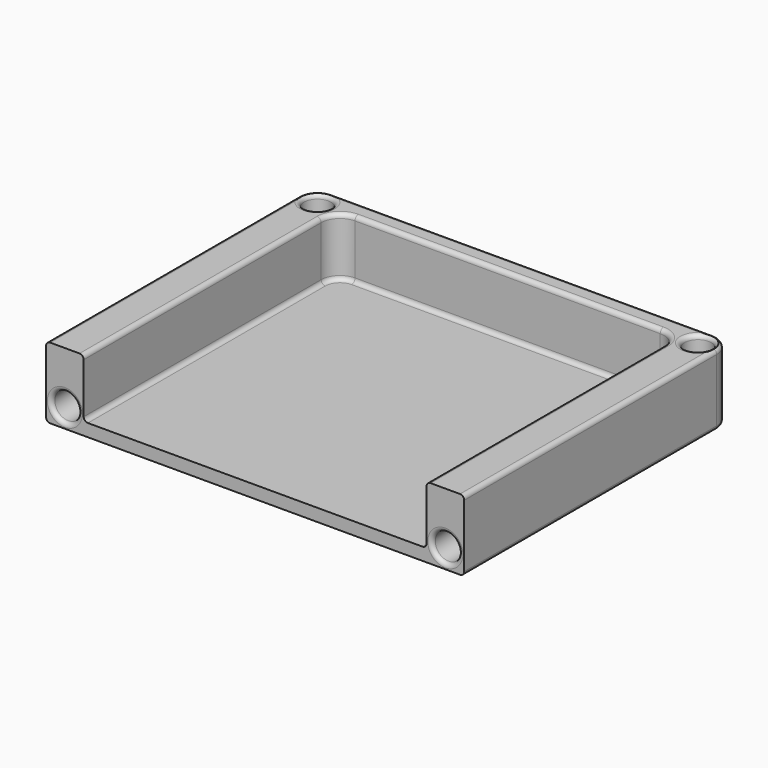
from build123d import *

# Parameters (mm, degrees)
F1_DEPTH     = 17
F5_DEPTH     = 14
F3_R         = 3.2
F6_DEPTH     = 10
F4_R         = 3.2
F7_DEPTH     = 10
F8_T1_DEPTH  = 73
F8_T3_DEPTH  = 71
F8_T6_ANGLE  = 90
F8_T8_ANGLE  = 90
F8_T9_DEPTH  = 78
F8_T11_DEPTH = 73.5
F8_T13_DEPTH = 73
F8_T15_DEPTH = 91
F8_T26_ANGLE = 90
F8_T28_ANGLE = 90
F8_T30_ANGLE = 90
F8_T32_ANGLE = 90
F8_T34_ANGLE = 90
F8_T36_ANGLE = 90


# Not quite as in the source:
# - a fillet or chamfer that OpenCascade refuses, or shapes differently, is made with other operations: its cross-section is extruded or revolved along the edge and cut away or added


with BuildPart() as f1:
    # F0 (on Top) → F1 (new body)
    with BuildSketch(Plane.XY):
        with BuildLine():
            Line((0, 75.5), (0, 0))
            Line((0, 0), (50, 0))
            Line((50, 0), (100, 0))
            Line((100, 0), (100, 75.5))
            ThreePointArc((100, 75.5), (98.6819805153, 78.6819805153), (95.5, 80))
            Line((95.5, 80), (50, 80))
            Line((50, 80), (4.5, 80))
            ThreePointArc((4.5, 80), (1.3180194847, 78.6819805153), (0, 75.5))
        make_face()
    extrude(amount=F1_DEPTH)

    # F3 (on offset) → F5 (cut)
    with BuildSketch(Plane.XY.offset(17)):
        with BuildLine():
            Line((9, 71), (9, 0))
            Line((9, 0), (50, 0))
            Line((50, 0), (91, 0))
            Line((91, 0), (91, 71))
            ThreePointArc((91, 71), (89.6819805153, 74.1819805153), (86.5, 75.5))
            Line((86.5, 75.5), (50, 75.5))
            Line((50, 75.5), (13.5, 75.5))
            ThreePointArc((13.5, 75.5), (10.3180194847, 74.1819805153), (9, 71))
        make_face()
    extrude(amount=-F5_DEPTH, mode=Mode.SUBTRACT)

    # F3 (on offset) → F6 (cut)
    with BuildSketch(Plane.XY.offset(17)):
        with Locations((4.5, 75.5)):
            Circle(F3_R)
        with Locations((95.5, 75.5)):
            Circle(F3_R)
    extrude(amount=-F6_DEPTH, mode=Mode.SUBTRACT)

    # F4 (on Front) → F7 (cut)
    with BuildSketch(Plane.XZ):
        with Locations((4.5, 4.5)):
            Circle(F4_R)
        with Locations((95.5, 4.5)):
            Circle(F4_R)
    extrude(amount=-F7_DEPTH, mode=Mode.SUBTRACT)

    # F8: fillet of radius 1 on 8 edges, made by hand

    # F8_s2 → F8_t1 (join)
    with BuildSketch(Plane.YZ.offset(13.5)):
        with BuildLine():
            ThreePointArc((74.5, 3), (75.2071067812, 3.2928932188), (75.5, 4))
            Line((75.5, 4), (75.5, 3))
            Line((75.5, 3), (74.5, 3))
        make_face()
    extrude(amount=F8_T1_DEPTH)

    # F8_s4 → F8_t3 (join)
    with BuildSketch(Plane.XZ.offset(-71)):
        with BuildLine():
            ThreePointArc((9, 4), (9.2928932188, 3.2928932188), (10, 3))
            Line((10, 3), (9, 3))
            Line((9, 3), (9, 4))
        make_face()
        with BuildLine():
            ThreePointArc((91, 4), (90.7071067812, 3.2928932188), (90, 3))
            Line((90, 3), (91, 3))
            Line((91, 3), (91, 4))
        make_face()
    extrude(amount=F8_T3_DEPTH)

    # F8_s5 → F8_t6 (revolve)
    with BuildSketch(Plane.XZ.offset(-71)):
        with BuildLine():
            ThreePointArc((90, 3), (90.7071067812, 3.2928932188), (91, 4))
            Line((91, 4), (91, 3))
            Line((91, 3), (90, 3))
        make_face()
    revolve(axis=Axis((86.5, 71, 3), (0, 0, 1)), revolution_arc=F8_T6_ANGLE)

    # F8_s7 → F8_t8 (revolve)
    with BuildSketch(Plane.YZ.offset(13.5)):
        with BuildLine():
            ThreePointArc((74.5, 3), (75.2071067812, 3.2928932188), (75.5, 4))
            Line((75.5, 4), (75.5, 3))
            Line((75.5, 3), (74.5, 3))
        make_face()
    revolve(axis=Axis((13.5, 71, 3), (0, 0, 1)), revolution_arc=F8_T8_ANGLE)

    # F8_s10 → F8_t9 (cut)
    with BuildSketch(Plane.XZ.offset(-75.5)):
        with BuildLine():
            ThreePointArc((99, 17), (99.7071067812, 16.7071067812), (100, 16))
            Line((100, 16), (100, 17))
            Line((100, 17), (99, 17))
        make_face()
        with BuildLine():
            ThreePointArc((99, 0), (99.7071067812, 0.2928932188), (100, 1))
            Line((100, 1), (100, 0))
            Line((100, 0), (99, 0))
        make_face()
        with BuildLine():
            ThreePointArc((0, 1), (0.2928932188, 0.2928932188), (1, 0))
            Line((1, 0), (0, 0))
            Line((0, 0), (0, 1))
        make_face()
        with BuildLine():
            ThreePointArc((0, 16), (0.2928932188, 16.7071067812), (1, 17))
            Line((1, 17), (0, 17))
            Line((0, 17), (0, 16))
        make_face()
    extrude(amount=F8_T9_DEPTH, mode=Mode.SUBTRACT)

    # F8_s12 → F8_t11 (cut)
    with BuildSketch(Plane.XZ.offset(-71)):
        with BuildLine():
            ThreePointArc((8, 17), (8.7071067812, 16.7071067812), (9, 16))
            Line((9, 16), (9, 17))
            Line((9, 17), (8, 17))
        make_face()
        with BuildLine():
            ThreePointArc((92, 17), (91.2928932188, 16.7071067812), (91, 16))
            Line((91, 16), (91, 17))
            Line((91, 17), (92, 17))
        make_face()
    extrude(amount=F8_T11_DEPTH, mode=Mode.SUBTRACT)

    # F8_s14 → F8_t13 (cut)
    with BuildSketch(Plane.YZ.offset(13.5)):
        with BuildLine():
            ThreePointArc((76.5, 17), (75.7928932188, 16.7071067812), (75.5, 16))
            Line((75.5, 16), (75.5, 17))
            Line((75.5, 17), (76.5, 17))
        make_face()
    extrude(amount=F8_T13_DEPTH, mode=Mode.SUBTRACT)

    # F8_s16 → F8_t15 (cut)
    with BuildSketch(Plane.YZ.offset(4.5)):
        with BuildLine():
            ThreePointArc((79, 0), (79.7071067812, 0.2928932188), (80, 1))
            Line((80, 1), (80, 0))
            Line((80, 0), (79, 0))
        make_face()
        with BuildLine():
            ThreePointArc((79, 17), (79.7071067812, 16.7071067812), (80, 16))
            Line((80, 16), (80, 17))
            Line((80, 17), (79, 17))
        make_face()
    extrude(amount=F8_T15_DEPTH, mode=Mode.SUBTRACT)

    # F8_s17 → F8_t18 (revolve, cut)
    with BuildSketch(Plane.XY.offset(4.5)):
        with BuildLine():
            ThreePointArc((8.7, 0), (7.9928932188, 0.2928932188), (7.7, 1))
            Line((7.7, 1), (7.7, 0))
            Line((7.7, 0), (8.7, 0))
        make_face()
    revolve(axis=Axis((4.5, 0, 4.5), (0, -1, 0)), mode=Mode.SUBTRACT)

    # F8_s19 → F8_t20 (revolve, cut)
    with BuildSketch(Plane.XY.offset(4.5)):
        with BuildLine():
            ThreePointArc((99.7, 0), (98.9928932188, 0.2928932188), (98.7, 1))
            Line((98.7, 1), (98.7, 0))
            Line((98.7, 0), (99.7, 0))
        make_face()
    revolve(axis=Axis((95.5, 0, 4.5), (0, -1, 0)), mode=Mode.SUBTRACT)

    # F8_s21 → F8_t22 (revolve, cut)
    with BuildSketch(Plane.XZ.offset(-75.5)):
        with BuildLine():
            ThreePointArc((99.7, 17), (98.9928932188, 16.7071067812), (98.7, 16))
            Line((98.7, 16), (98.7, 17))
            Line((98.7, 17), (99.7, 17))
        make_face()
    revolve(axis=Axis((95.5, 75.5, 17), (0, 0, 1)), mode=Mode.SUBTRACT)

    # F8_s23 → F8_t24 (revolve, cut)
    with BuildSketch(Plane.XZ.offset(-75.5)):
        with BuildLine():
            ThreePointArc((8.7, 17), (7.9928932188, 16.7071067812), (7.7, 16))
            Line((7.7, 16), (7.7, 17))
            Line((7.7, 17), (8.7, 17))
        make_face()
    revolve(axis=Axis((4.5, 75.5, 17), (0, 0, 1)), mode=Mode.SUBTRACT)

    # F8_s25 → F8_t26 (revolve, cut)
    with BuildSketch(Plane.YZ.offset(13.5)):
        with BuildLine():
            ThreePointArc((76.5, 17), (75.7928932188, 16.7071067812), (75.5, 16))
            Line((75.5, 16), (75.5, 17))
            Line((75.5, 17), (76.5, 17))
        make_face()
    revolve(axis=Axis((13.5, 71, 17), (0, 0, 1)), revolution_arc=F8_T26_ANGLE, mode=Mode.SUBTRACT)

    # F8_s27 → F8_t28 (revolve, cut)
    with BuildSketch(Plane.XZ.offset(-71)):
        with BuildLine():
            ThreePointArc((92, 17), (91.2928932188, 16.7071067812), (91, 16))
            Line((91, 16), (91, 17))
            Line((91, 17), (92, 17))
        make_face()
    revolve(axis=Axis((86.5, 71, 17), (0, 0, 1)), revolution_arc=F8_T28_ANGLE, mode=Mode.SUBTRACT)

    # F8_s29 → F8_t30 (revolve, cut)
    with BuildSketch(Plane.XZ.offset(-75.5)):
        with BuildLine():
            ThreePointArc((99, 0), (99.7071067812, 0.2928932188), (100, 1))
            Line((100, 1), (100, 0))
            Line((100, 0), (99, 0))
        make_face()
    revolve(axis=Axis((95.5, 75.5, 0), (0, 0, 1)), revolution_arc=F8_T30_ANGLE, mode=Mode.SUBTRACT)

    # F8_s31 → F8_t32 (revolve, cut)
    with BuildSketch(Plane.YZ.offset(4.5)):
        with BuildLine():
            ThreePointArc((80, 1), (79.7071067812, 0.2928932188), (79, 0))
            Line((79, 0), (80, 0))
            Line((80, 0), (80, 1))
        make_face()
    revolve(axis=Axis((4.5, 75.5, 0), (0, 0, 1)), revolution_arc=F8_T32_ANGLE, mode=Mode.SUBTRACT)

    # F8_s33 → F8_t34 (revolve, cut)
    with BuildSketch(Plane.XZ.offset(-75.5)):
        with BuildLine():
            ThreePointArc((99, 17), (99.7071067812, 16.7071067812), (100, 16))
            Line((100, 16), (100, 17))
            Line((100, 17), (99, 17))
        make_face()
    revolve(axis=Axis((95.5, 75.5, 17), (0, 0, 1)), revolution_arc=F8_T34_ANGLE, mode=Mode.SUBTRACT)

    # F8_s35 → F8_t36 (revolve, cut)
    with BuildSketch(Plane.YZ.offset(4.5)):
        with BuildLine():
            ThreePointArc((80, 16), (79.7071067812, 16.7071067812), (79, 17))
            Line((79, 17), (80, 17))
            Line((80, 17), (80, 16))
        make_face()
    revolve(axis=Axis((4.5, 75.5, 17), (0, 0, 1)), revolution_arc=F8_T36_ANGLE, mode=Mode.SUBTRACT)


solid = f1.part
